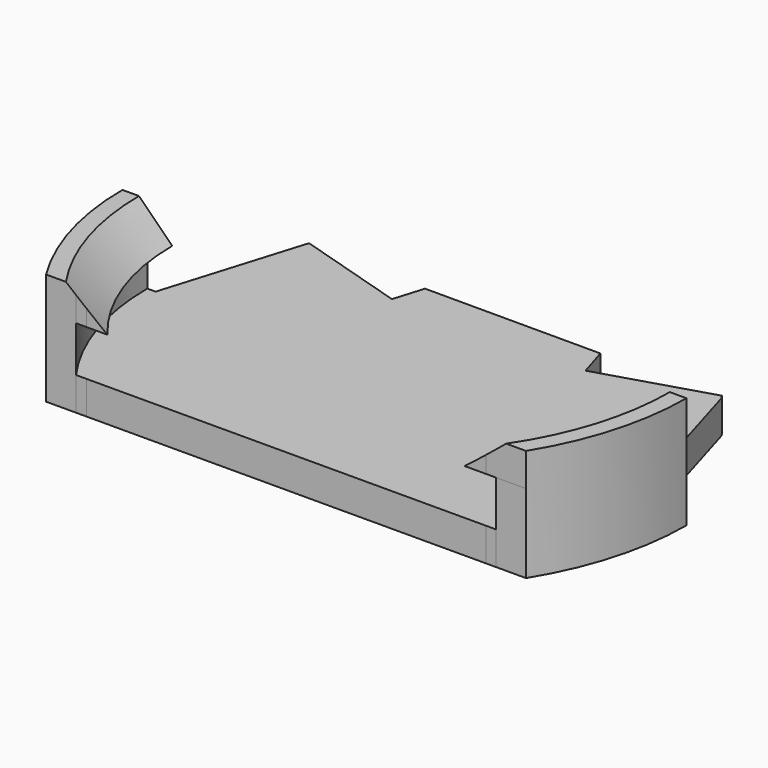
from build123d import *

# Parameters (mm, degrees)
F2_DEPTH    = 2
F4_DEPTH    = 2.75
F6_DEPTH    = 2
F7_T2_ANGLE = 111.7162943046
F7_T4_ANGLE = 111.4349059649


# Not quite as in the source:
# - a fillet or chamfer that OpenCascade refuses, or shapes differently, is made with other operations: its cross-section is extruded or revolved along the edge and cut away or added


with BuildPart() as f2:
    # F1 (on Top) → F2 (new body)
    with BuildSketch(Plane.XY):
        with BuildLine():
            ThreePointArc((-12.615433857, -11.3439912447), (-14.7570217863, -7.0788626246), (-15.4994493417, -2.3643613435))
            Line((-15.4994493417, -2.3643613435), (-16.9994473669, -2.3667953738))
            ThreePointArc((-16.9994473669, -2.3667953738), (-16.3370166369, -7.0385981193), (-14.4159247362, -11.34835))
            Line((-14.4159247362, -11.34835), (-12.615433857, -11.3439912447))
        make_face()
        with BuildLine():
            ThreePointArc((-11.9969468723, -11.3424939678), (-14.2251992258, -7.0961265352), (-14.99945, -2.36355))
            Line((-14.99945, -2.36355), (-15.4994493417, -2.3643613435))
            ThreePointArc((-15.4994493417, -2.3643613435), (-14.7570217863, -7.0788626246), (-12.615433857, -11.3439912447))
            Line((-12.615433857, -11.3439912447), (-11.9969468723, -11.3424939678))
        make_face()
        with BuildLine():
            Line((-12.44455, 6.00525), (-14.99945, -2.36355))
            ThreePointArc((-14.99945, -2.36355), (-14.2251992258, -7.0961265352), (-11.9969468723, -11.3424939678))
            Line((-11.9969468723, -11.3424939678), (12.0415, -11.2843))
            ThreePointArc((12.0415, -11.2843), (14.2377010351, -7.0616579823), (15.00045, -2.36355))
            Line((15.00045, -2.36355), (12.58545, 5.79585))
            Line((12.58545, 5.79585), (12.44455, 6.00525))
            Line((12.44455, 6.00525), (5.8368961963, 3.9880080175))
            Line((5.8368961963, 3.9880080175), (5.2849824833, 5.79585))
            Line((5.2849824833, 5.79585), (0, 5.79585))
            Line((0, 5.79585), (-5.2849824833, 5.79585))
            Line((-5.2849824833, 5.79585), (-5.8368961963, 3.9880080175))
            Line((-5.8368961963, 3.9880080175), (-12.44455, 6.00525))
        make_face()
        with BuildLine():
            ThreePointArc((15.00045, -2.36355), (14.2377010351, -7.0616579823), (12.0415, -11.2843))
            Line((12.0415, -11.2843), (12.6599780988, -11.2828027446))
            ThreePointArc((12.6599780988, -11.2828027446), (14.7694777267, -7.043108573), (15.5004493418, -2.3643613211))
            Line((15.5004493418, -2.3643613211), (15.00045, -2.36355))
        make_face()
        with BuildLine():
            ThreePointArc((15.5004493418, -2.3643613211), (14.7694777267, -7.043108573), (12.6599780988, -11.2828027446))
            Line((12.6599780988, -11.2828027446), (14.4604487154, -11.2784440383))
            ThreePointArc((14.4604487154, -11.2784440383), (16.3493648109, -6.9990233555), (17.000447367, -2.3667952845))
            Line((17.000447367, -2.3667952845), (15.5004493418, -2.3643613211))
        make_face()
    extrude(amount=F2_DEPTH)

    # F3 (on face) → F4 (join)
    with BuildSketch(Plane.XY.offset(2)):
        with BuildLine():
            ThreePointArc((-12.615433857, -11.3439912447), (-14.7570217863, -7.0788626246), (-15.4994493417, -2.3643613435))
            Line((-15.4994493417, -2.3643613435), (-16.9994473669, -2.3667953738))
            ThreePointArc((-16.9994473669, -2.3667953738), (-16.3370166369, -7.0385981193), (-14.4159247362, -11.34835))
            Line((-14.4159247362, -11.34835), (-12.615433857, -11.3439912447))
        make_face()
        with BuildLine():
            ThreePointArc((15.5004493418, -2.3643613211), (14.7694777267, -7.043108573), (12.6599780988, -11.2828027446))
            Line((12.6599780988, -11.2828027446), (14.4604487154, -11.2784440383))
            ThreePointArc((14.4604487154, -11.2784440383), (16.3493648109, -6.9990233555), (17.000447367, -2.3667952845))
            Line((17.000447367, -2.3667952845), (15.5004493418, -2.3643613211))
        make_face()
    extrude(amount=F4_DEPTH)

    # F5 (on face) → F6 (join)
    with BuildSketch(Plane.XY.offset(4.75)):
        with BuildLine():
            ThreePointArc((-11.9969468723, -11.3424939678), (-14.2251992258, -7.0961265352), (-14.99945, -2.36355))
            Line((-14.99945, -2.36355), (-15.4994493417, -2.3643613435))
            ThreePointArc((-15.4994493417, -2.3643613435), (-14.7570217863, -7.0788626246), (-12.615433857, -11.3439912447))
            Line((-12.615433857, -11.3439912447), (-11.9969468723, -11.3424939678))
        make_face()
        with BuildLine():
            ThreePointArc((-12.615433857, -11.3439912447), (-14.7570217863, -7.0788626246), (-15.4994493417, -2.3643613435))
            Line((-15.4994493417, -2.3643613435), (-16.9994473669, -2.3667953738))
            ThreePointArc((-16.9994473669, -2.3667953738), (-16.3370166369, -7.0385981193), (-14.4159247362, -11.34835))
            Line((-14.4159247362, -11.34835), (-12.615433857, -11.3439912447))
        make_face()
        with BuildLine():
            Line((-12.9994526331, -2.3603046262), (-14.99945, -2.36355))
            ThreePointArc((-14.99945, -2.36355), (-14.2251992258, -7.0961265352), (-11.9969468723, -11.3424939678))
            Line((-11.9969468723, -11.3424939678), (-9.3831293237, -11.3361662539))
            ThreePointArc((-9.3831293237, -11.3361662539), (-12.0576120471, -7.1972712434), (-12.9994526331, -2.3603046262))
        make_face()
        with BuildLine():
            ThreePointArc((13.000452633, -2.3603047155), (12.0703811691, -7.1680366652), (9.4277378752, -11.2906275797))
            Line((9.4277378752, -11.2906275797), (12.0415, -11.2843))
            ThreePointArc((12.0415, -11.2843), (14.2377010351, -7.0616579823), (15.00045, -2.36355))
            Line((15.00045, -2.36355), (13.000452633, -2.3603047155))
        make_face()
        with BuildLine():
            ThreePointArc((15.00045, -2.36355), (14.2377010351, -7.0616579823), (12.0415, -11.2843))
            Line((12.0415, -11.2843), (14.4604487154, -11.2784440383))
            ThreePointArc((14.4604487154, -11.2784440383), (16.3493648109, -6.9990233555), (17.000447367, -2.3667952845))
            Line((17.000447367, -2.3667952845), (15.00045, -2.36355))
        make_face()
    extrude(amount=F6_DEPTH)

    # F7: chamfer of 3 on 2 edges, made by hand

    # F7_s1 → F7_t2 (revolve, cut)
    with BuildSketch(Plane(origin=(0.4833612439, -0.1044854652, 0), x_dir=(0, 0, 1), z_dir=(0.9774246375, -0.2112843535, 0))):
        Polygon((3.75, 15.2861027758), (6.75, 18.2861027758), (6.75, 15.2861027758), align=None)
    revolve(axis=Axis((0.0002934681, -2.3392100804, 6.75), (0, 0, -1)), revolution_arc=F7_T2_ANGLE, mode=Mode.SUBTRACT)

    # F7_s3 → F7_t4 (revolve, cut)
    with BuildSketch(Plane(origin=(1.0831916717, -1.6111813469, 0), x_dir=(0, 0, 1), z_dir=(-0.5579305881, 0.8298876182, 0))):
        Polygon((6.75, 14.695302969), (3.75, 11.695302969), (6.75, 11.695302969), align=None)
    revolve(axis=Axis((0.0002934681, -2.3392100804, 6.75), (0, 0, -1)), revolution_arc=F7_T4_ANGLE, mode=Mode.SUBTRACT)


solid = f2.part
